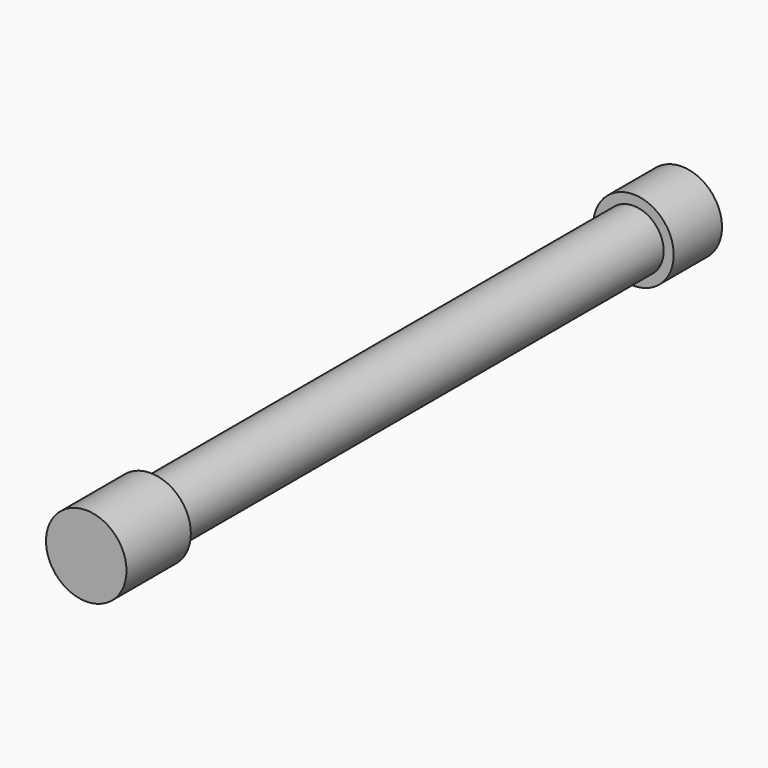
from build123d import *

# Parameters (mm, degrees)
F0_R     = 3
F1_DEPTH = 30
F3_R     = 4
F3_R_2   = 3
F4_DEPTH = 6
F2_R     = 4
F2_R_2   = 3
F5_DEPTH = 8


with BuildPart() as f1:
    # F0 (on Front) → F1 (new body, symmetric)
    with BuildSketch(Plane.XZ):
        Circle(F0_R)
    extrude(amount=F1_DEPTH, both=True)

    # F3 (on face) → F4 (join)
    with BuildSketch(Plane(origin=(0, 30, 0), x_dir=(-1, 0, 0), z_dir=(0, 1, 0))):
        Circle(F3_R)
        Circle(F3_R_2, mode=Mode.SUBTRACT)
        Circle(F3_R_2)
    extrude(amount=F4_DEPTH)

    # F2 (on face) → F5 (join)
    with BuildSketch(Plane.XZ.offset(30)):
        Circle(F2_R)
        Circle(F2_R_2, mode=Mode.SUBTRACT)
        Circle(F2_R_2)
    extrude(amount=F5_DEPTH)


solid = f1.part
